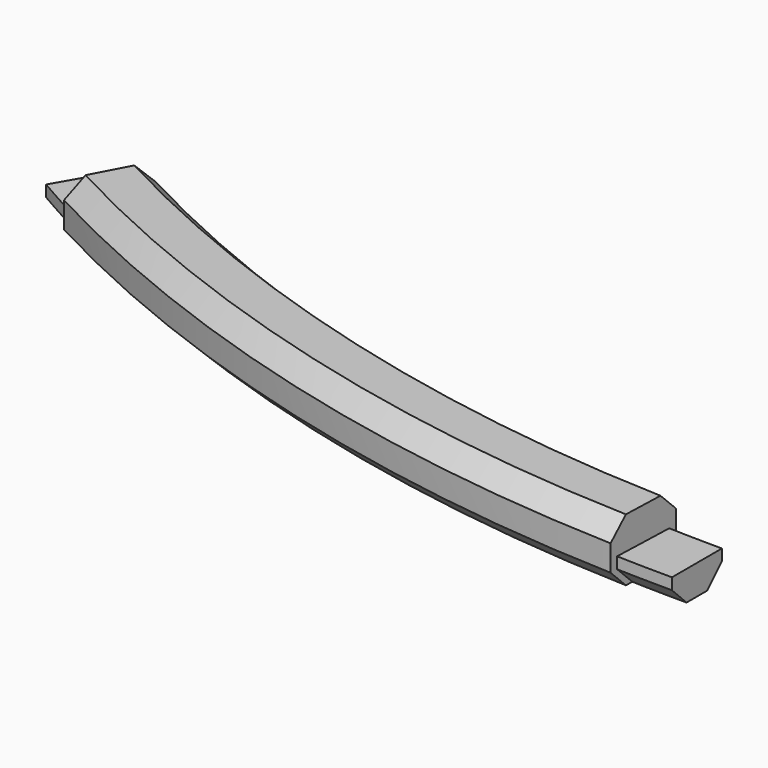
from build123d import *

# Parameters (mm, degrees)
F3_ANGLE_BACK = 15
F3_ANGLE      = 30
F4_ANGLE_BACK = 13
F4_ANGLE      = 26
F5_ANGLE      = 15


# Not quite as in the source:
# - a feature of the source that left no trace in its solid (it failed there, or was rolled back) is left out


with BuildPart() as f3:
    # F0 (on Right) → F3 (revolve)
    with BuildSketch(Plane.YZ, mode=Mode.PRIVATE) as f3_sk:
        Polygon((-198.3431457505, -4), (-196, -1.6568542495), (-196, -0.2), (-204, -0.2), (-204, -1.6568542495), (-201.6568542495, -4), align=None)
    revolve(f3_sk.sketch.rotate(Axis((0, 0, 14.9391144514), (0, 0, -1)), -F3_ANGLE_BACK), axis=Axis((0, 0, 14.9391144514), (0, 0, -1)), revolution_arc=F3_ANGLE)

    # F2 (on Right) → F4 (revolve)
    with BuildSketch(Plane.YZ, mode=Mode.PRIVATE) as f4_sk:
        Polygon((-195, 1.6568542495), (-197.3431457505, 4), (-202.6568542495, 4), (-205, 1.6568542495), (-205, -1.6568542495), (-202.6568542495, -4), (-197.3431457505, -4), (-195, -1.6568542495), align=None)
    revolve(f4_sk.sketch.rotate(Axis((0, 0, 27.1144676954), (0, 0, 1)), -F4_ANGLE_BACK), axis=Axis((0, 0, 27.1144676954), (0, 0, 1)), revolution_arc=F4_ANGLE)


with BuildPart() as f3_1:
    # F5: moved
    add(f3.part.rotate(Axis((0, 0, 14.9391144514), (0, 0, -1)), F5_ANGLE))


solid = f3_1.part
